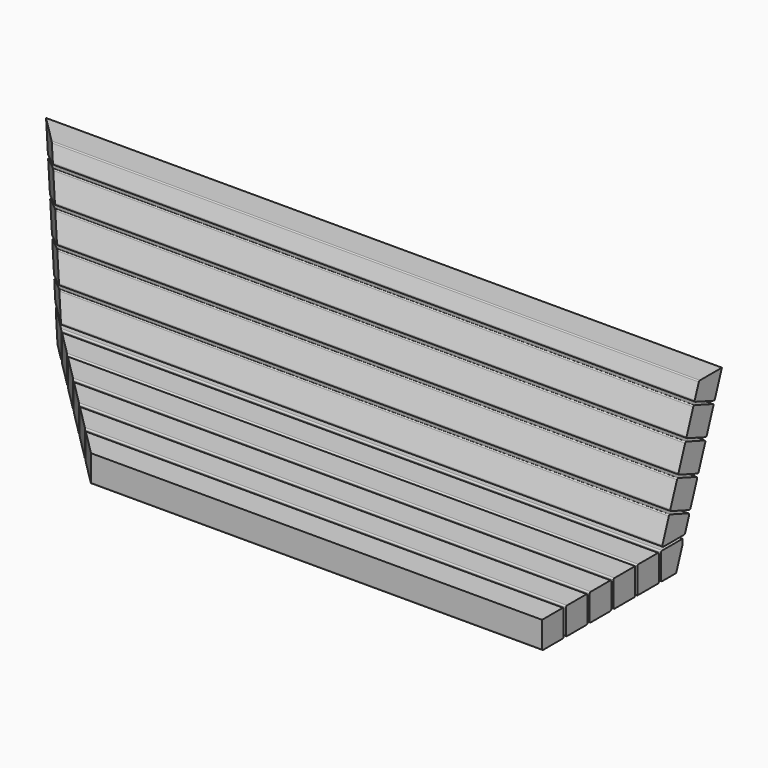
from build123d import *

# Parameters (mm, degrees)
F1_DEPTH = 2500
F3_DEPTH = 583.2330008918


# Not quite as in the source:
# - a feature names something its author has since deleted; it is built from what else it names


with BuildPart() as f1:
    # F0 (on Right) → F1 (new body)
    with BuildSketch(Plane.YZ):
        with BuildLine():
            Line((0, -16.7510631673), (0, 0))
            Line((0, 0), (-95, 0))
            ThreePointArc((-95, 0), (-98.5355339059, -1.4644660941), (-100, -5))
            Line((-100, -5), (-100, -95))
            ThreePointArc((-100, -95), (-98.5355339059, -98.5355339059), (-95, -100))
            Line((-95, -100), (-33.4802838701, -100))
            ThreePointArc((-33.4802838701, -100), (-30.6124016883, -99.0957602214), (-28.7818207661, -96.7101007166))
            Line((-28.7818207661, -96.7101007166), (-0.3015368961, -18.4611638839))
            ThreePointArc((-0.3015368961, -18.4611638839), (-0.0759612349, -17.6193040556), (0, -16.7510631673))
        make_face()
    extrude(amount=F1_DEPTH)


with BuildPart() as f1b:
    # F0 (on Right) → F1, piece 2 (new body)
    with BuildSketch(Plane.YZ):
        with BuildLine():
            ThreePointArc((-110, -5), (-111.4644660941, -1.4644660941), (-115, 0))
            Line((-115, 0), (-205, 0))
            ThreePointArc((-205, 0), (-208.5355339059, -1.4644660941), (-210, -5))
            Line((-210, -5), (-210, -100))
            Line((-210, -100), (-115, -100))
            ThreePointArc((-115, -100), (-111.4644660941, -98.5355339059), (-110, -95))
            Line((-110, -95), (-110, -5))
        make_face()
    extrude(amount=F1_DEPTH)


with BuildPart() as f1c:
    # F0 (on Right) → F1, piece 3 (new body)
    with BuildSketch(Plane.YZ):
        with BuildLine():
            Line((-220, -95), (-220, 0))
            Line((-220, 0), (-315, 0))
            ThreePointArc((-315, 0), (-318.5355339059, -1.4644660941), (-320, -5))
            Line((-320, -5), (-320, -95))
            ThreePointArc((-320, -95), (-318.5355339059, -98.5355339059), (-315, -100))
            Line((-315, -100), (-225, -100))
            ThreePointArc((-225, -100), (-221.4644660941, -98.5355339059), (-220, -95))
        make_face()
    extrude(amount=F1_DEPTH)


with BuildPart() as f1d:
    # F0 (on Right) → F1, piece 4 (new body)
    with BuildSketch(Plane.YZ):
        with BuildLine():
            ThreePointArc((-330, -5), (-331.4644660941, -1.4644660941), (-335, 0))
            Line((-335, 0), (-425, 0))
            ThreePointArc((-425, 0), (-428.5355339059, -1.4644660941), (-430, -5))
            Line((-430, -5), (-430, -95))
            ThreePointArc((-430, -95), (-428.5355339059, -98.5355339059), (-425, -100))
            Line((-425, -100), (-335, -100))
            ThreePointArc((-335, -100), (-331.4644660941, -98.5355339059), (-330, -95))
            Line((-330, -95), (-330, -5))
        make_face()
    extrude(amount=F1_DEPTH)


with BuildPart() as f1e:
    # F0 (on Right) → F1, piece 5 (new body)
    with BuildSketch(Plane.YZ):
        with BuildLine():
            ThreePointArc((-440, -5), (-441.4644660941, -1.4644660941), (-445, 0))
            Line((-445, 0), (-535, 0))
            ThreePointArc((-535, 0), (-538.5355339059, -1.4644660941), (-540, -5))
            Line((-540, -5), (-540, -95))
            ThreePointArc((-540, -95), (-538.5355339059, -98.5355339059), (-535, -100))
            Line((-535, -100), (-445, -100))
            ThreePointArc((-445, -100), (-441.4644660941, -98.5355339059), (-440, -95))
            Line((-440, -95), (-440, -5))
        make_face()
    extrude(amount=F1_DEPTH)


with BuildPart() as f1f:
    # F0 (on Right) → F1, piece 6 (new body)
    with BuildSketch(Plane.YZ):
        with BuildLine():
            ThreePointArc((-550, -5), (-551.4644660941, -1.4644660941), (-555, 0))
            Line((-555, 0), (-650, 0))
            Line((-650, 0), (-650, -95))
            ThreePointArc((-650, -95), (-648.5355339059, -98.5355339059), (-645, -100))
            Line((-645, -100), (-555, -100))
            ThreePointArc((-555, -100), (-551.4644660941, -98.5355339059), (-550, -95))
            Line((-550, -95), (-550, -5))
        make_face()
    extrude(amount=F1_DEPTH)


with BuildPart() as f1g:
    # F0 (on Right) → F1, piece 7 (new body)
    with BuildSketch(Plane.YZ):
        with BuildLine():
            Line((-63.8683840414, 99.2707989747), (-93.9180207276, 16.7101007166))
            ThreePointArc((-93.9180207276, 16.7101007166), (-93.3153178451, 12.1321178182), (-89.2195576236, 10))
            Line((-89.2195576236, 10), (6.5564418992, 10))
            ThreePointArc((6.5564418992, 10), (9.424324081, 10.9042397786), (11.2549050031, 13.2898992834))
            Line((11.2549050031, 13.2898992834), (30.1008780372, 65.0687846421))
            ThreePointArc((30.1008780372, 65.0687846421), (29.9339538684, 68.8919766674), (27.1125156499, 71.4773484627))
            Line((27.1125156499, 71.4773484627), (-57.4598202208, 102.259161362))
            ThreePointArc((-57.4598202208, 102.259161362), (-61.2830122462, 102.0922371932), (-63.8683840414, 99.2707989747))
        make_face()
    extrude(amount=F1_DEPTH)


with BuildPart() as f1h:
    # F0 (on Right) → F1, piece 8 (new body)
    with BuildSketch(Plane.YZ):
        with BuildLine():
            ThreePointArc((-57.0279811749, 118.0646513904), (-56.8610570061, 114.241459365), (-54.0396187876, 111.6560875698))
            Line((-54.0396187876, 111.6560875698), (29.8241305782, 81.1321790667))
            ThreePointArc((29.8241305782, 81.1321790667), (33.6473226035, 81.2991032355), (36.2326943987, 84.120541454))
            Line((36.2326943987, 84.120541454), (67.014507298, 168.6928773248))
            ThreePointArc((67.014507298, 168.6928773248), (66.8475831293, 172.5160693501), (64.0261449107, 175.1014411453))
            Line((64.0261449107, 175.1014411453), (-19.837604455, 205.6253496484))
            ThreePointArc((-19.837604455, 205.6253496484), (-23.6607964803, 205.4584254797), (-26.2461682756, 202.6369872611))
            Line((-26.2461682756, 202.6369872611), (-57.0279811749, 118.0646513904))
        make_face()
    extrude(amount=F1_DEPTH)


with BuildPart() as f1i:
    # F0 (on Right) → F1, piece 9 (new body)
    with BuildSketch(Plane.YZ):
        with BuildLine():
            Line((11.3760474902, 306.0031755476), (-19.4057654091, 221.4308396768))
            ThreePointArc((-19.4057654091, 221.4308396768), (-19.2388412403, 217.6076476515), (-16.4174030218, 215.0222758563))
            Line((-16.4174030218, 215.0222758563), (67.446346344, 184.4983673532))
            ThreePointArc((67.446346344, 184.4983673532), (71.2695383693, 184.6652915219), (73.8549101645, 187.4867297405))
            Line((73.8549101645, 187.4867297405), (104.6367230638, 272.0590656112))
            ThreePointArc((104.6367230638, 272.0590656112), (104.4697988951, 275.8822576365), (101.6483606765, 278.4676294318))
            Line((101.6483606765, 278.4676294318), (17.7846113108, 308.9915379349))
            ThreePointArc((17.7846113108, 308.9915379349), (13.9614192855, 308.8246137661), (11.3760474902, 306.0031755476))
        make_face()
    extrude(amount=F1_DEPTH)


with BuildPart() as f1j:
    # F0 (on Right) → F1, piece 10 (new body)
    with BuildSketch(Plane.YZ):
        with BuildLine():
            Line((149.0993416962, 394.2191063134), (181.4973857886, 483.2320008918))
            Line((181.4973857886, 483.2320008918), (79.3831022606, 483.2320008918))
            ThreePointArc((79.3831022606, 483.2320008918), (76.5152200788, 482.3277611133), (74.6846391566, 479.9421016085))
            Line((74.6846391566, 479.9421016085), (55.8386661226, 428.1632162497))
            ThreePointArc((55.8386661226, 428.1632162497), (56.0055902913, 424.3400242244), (58.8270285099, 421.7546524292))
            Line((58.8270285099, 421.7546524292), (142.6907778756, 391.2307439261))
            ThreePointArc((142.6907778756, 391.2307439261), (146.513969901, 391.3976680948), (149.0993416962, 394.2191063134))
        make_face()
    extrude(amount=F1_DEPTH)


with BuildPart() as f1k:
    # F0 (on Right) → F1, piece 11 (new body)
    with BuildSketch(Plane.YZ):
        with BuildLine():
            ThreePointArc((18.2164503568, 324.7970279633), (18.3833745255, 320.9738359379), (21.2048127441, 318.3884641427))
            Line((21.2048127441, 318.3884641427), (105.0685621098, 287.8645556396))
            ThreePointArc((105.0685621098, 287.8645556396), (108.8917541351, 288.0314798084), (111.4771259304, 290.8529180269))
            Line((111.4771259304, 290.8529180269), (142.2589388297, 375.4252538977))
            ThreePointArc((142.2589388297, 375.4252538977), (142.0920146609, 379.248445923), (139.2705764424, 381.8338177182))
            Line((139.2705764424, 381.8338177182), (55.4068270766, 412.3577262213))
            ThreePointArc((55.4068270766, 412.3577262213), (51.5836350513, 412.1908020526), (48.9982632561, 409.369363834))
            Line((48.9982632561, 409.369363834), (18.2164503568, 324.7970279633))
        make_face()
    extrude(amount=F1_DEPTH)


with BuildPart() as f3_tool:
    # F2 (on face) → F3 (new body, through all)
    with BuildSketch(Plane.XY.offset(483.2320008918)):
        Polygon((0, 181.4973857886), (0, 79.3831022606), (102.114283528, 79.3831022606), align=None)
        Polygon((0, 79.3831022606), (0, -651.0000042114), (832.49739, -651.0000042114), (102.114283528, 79.3831022606), align=None)
    extrude(amount=-F3_DEPTH)


with BuildPart() as f1_1:
    add(f1.part)

    # F3: cut by f3_tool
    add(f3_tool.part, mode=Mode.SUBTRACT)


with BuildPart() as f1b_1:
    add(f1b.part)

    # F3: cut by f3_tool
    add(f3_tool.part, mode=Mode.SUBTRACT)


with BuildPart() as f1c_1:
    add(f1c.part)

    # F3: cut by f3_tool
    add(f3_tool.part, mode=Mode.SUBTRACT)


with BuildPart() as f1d_1:
    add(f1d.part)

    # F3: cut by f3_tool
    add(f3_tool.part, mode=Mode.SUBTRACT)


with BuildPart() as f1e_1:
    add(f1e.part)

    # F3: cut by f3_tool
    add(f3_tool.part, mode=Mode.SUBTRACT)


with BuildPart() as f1f_1:
    add(f1f.part)

    # F3: cut by f3_tool
    add(f3_tool.part, mode=Mode.SUBTRACT)


with BuildPart() as f1g_1:
    add(f1g.part)

    # F3: cut by f3_tool
    add(f3_tool.part, mode=Mode.SUBTRACT)


with BuildPart() as f1h_1:
    add(f1h.part)

    # F3: cut by f3_tool
    add(f3_tool.part, mode=Mode.SUBTRACT)


with BuildPart() as f1i_1:
    add(f1i.part)

    # F3: cut by f3_tool
    add(f3_tool.part, mode=Mode.SUBTRACT)


with BuildPart() as f1j_1:
    add(f1j.part)

    # F3: cut by f3_tool
    add(f3_tool.part, mode=Mode.SUBTRACT)


with BuildPart() as f1k_1:
    add(f1k.part)

    # F3: cut by f3_tool
    add(f3_tool.part, mode=Mode.SUBTRACT)


solid = Compound([f1_1.part, f1b_1.part, f1c_1.part, f1d_1.part, f1e_1.part, f1f_1.part, f1g_1.part, f1h_1.part, f1i_1.part, f1j_1.part, f1k_1.part])
